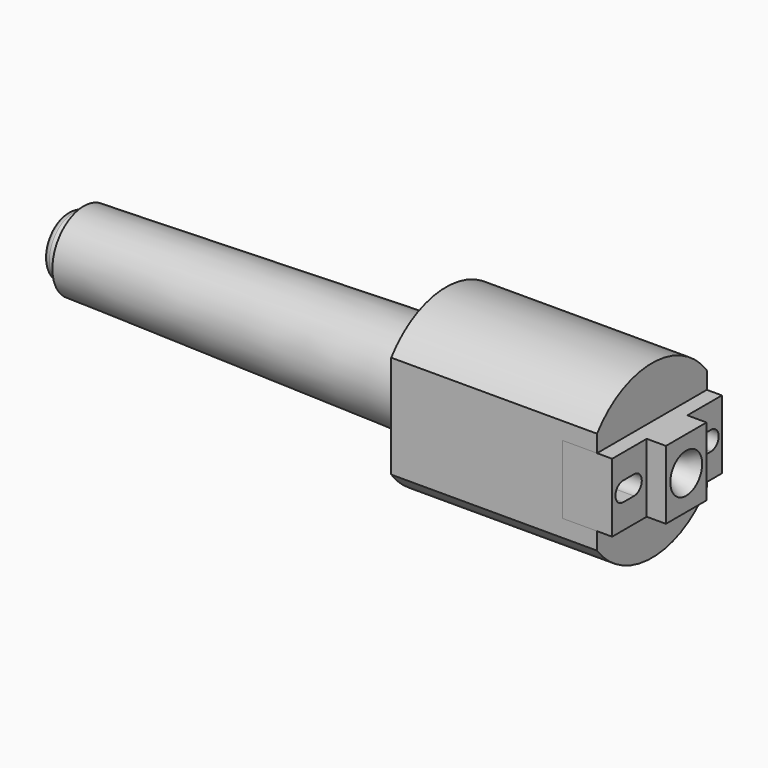
from build123d import *

# Parameters (mm, degrees)
F2_W      = 6.35
F2_H      = 12.7
F3_DEPTH  = 25.4
F6_DEPTH  = 38.1
F8_D      = 2.7051
F8_DEPTH  = 19.05
F8_TIP    = 0.8126940303
F9_DEPTH  = 12.7
F11_DEPTH = 25.4
F13_W     = 8.001
F13_H     = 12.7
F14_DEPTH = 3.556


# Not quite as in the source:
# - a feature names something its author has since deleted; it is built from what else it names


with BuildPart() as f1:
    # F0 (on Front) → F1 (revolve)
    with BuildSketch(Plane.XZ):
        Polygon((0, 5.588), (0, 0), (65.024, 0), (65.024, 8.89), (0, 7.2659854949), align=None)
        with BuildLine():
            Line((-3.175, 0), (0, 0))
            Line((0, 0), (0, 5.588))
            Line((0, 5.588), (-1.905, 5.588))
            ThreePointArc((-1.905, 5.588), (-2.8030256121, 5.2160256121), (-3.175, 4.318))
            Line((-3.175, 4.318), (-3.175, 0))
        make_face()
        with BuildLine():
            Line((65.024, 8.89), (65.024, 0))
            Line((65.024, 0), (67.056, 0))
            Line((67.056, 0), (67.056, 8.89))
            ThreePointArc((67.056, 8.89), (66.04, 8.5019225326), (65.024, 8.89))
        make_face()
        with BuildLine():
            Line((67.056, 8.89), (67.056, 0))
            Line((67.056, 0), (105.156, 0))
            Line((105.156, 0), (105.156, 15.875))
            Line((105.156, 15.875), (67.056, 15.875))
            Line((67.056, 15.875), (67.056, 11.1618450651))
            ThreePointArc((67.056, 11.1618450651), (67.4312152961, 10.6480929272), (67.564, 10.0259225326))
            ThreePointArc((67.564, 10.0259225326), (67.4312152961, 9.4037521379), (67.056, 8.89))
        make_face()
        with BuildLine():
            Line((67.056, 11.1618450651), (67.056, 8.89))
            ThreePointArc((67.056, 8.89), (67.4312152961, 9.4037521379), (67.564, 10.0259225326))
            ThreePointArc((67.564, 10.0259225326), (67.4312152961, 10.6480929272), (67.056, 11.1618450651))
        make_face()
    revolve(axis=Axis((32.512, 0, 0), (1, 0, 0)))

    # F2 (on Front) → F3 (cut, symmetric)
    with BuildSketch(Plane.XZ):
        with Locations((101.981, 0)):
            Rectangle(F2_W, F2_H)
    extrude(amount=F3_DEPTH, both=True, mode=Mode.SUBTRACT)

    # F4 (on face) → F6 (cut)
    with BuildSketch(Plane.YZ.offset(105.156)):
        with BuildLine():
            Line((-12.7, 6.35), (-14.5496778315, 6.35))
            ThreePointArc((-14.5496778315, 6.35), (-15.875, 0), (-14.5496778315, -6.35))
            ThreePointArc((-14.5496778315, -6.35), (-13.7170110348, -7.9911972363), (-12.7, -9.525))
            Line((-12.7, -9.525), (-12.7, 6.35))
        make_face()
        with BuildLine():
            ThreePointArc((-12.7, 9.525), (-13.7170110348, 7.9911972363), (-14.5496778315, 6.35))
            Line((-14.5496778315, 6.35), (-12.7, 6.35))
            Line((-12.7, 6.35), (-12.7, 9.525))
        make_face()
        with BuildLine():
            Line((14.5496778315, 6.35), (12.7, 6.35))
            Line((12.7, 6.35), (12.7, -9.525))
            ThreePointArc((12.7, -9.525), (13.7170110348, -7.9911972363), (14.5496778315, -6.35))
            ThreePointArc((14.5496778315, -6.35), (15.875, 0), (14.5496778315, 6.35))
        make_face()
        with BuildLine():
            Line((12.7, 9.525), (12.7, 6.35))
            Line((12.7, 6.35), (14.5496778315, 6.35))
            ThreePointArc((14.5496778315, 6.35), (13.7170110348, 7.9911972363), (12.7, 9.525))
        make_face()
    extrude(amount=-F6_DEPTH, mode=Mode.SUBTRACT)

    # F8
    with Locations(Plane.YZ.offset(98.806)):
        with Locations((-8.89, 0), (8.89, 0)):
            Hole(F8_D / 2, depth=F8_DEPTH)
            with Locations((0, 0, -(F8_DEPTH + F8_TIP / 2))):  # 118° drill point
                Cone(0, F8_D / 2, F8_TIP, mode=Mode.SUBTRACT)


with BuildPart() as f9:
    # F5 (on Front) → F9 (new body, symmetric)
    with BuildSketch(Plane.XZ):
        Polygon((98.806, 6.35), (98.806, -6.35), (111.506, -6.35), (111.506, -3.683), (111.506, 0), (103.9612241254, 0), (104.7014875327, 1.5875), (107.8764875327, 1.5875), (111.506, 3.683), (111.506, 6.35), align=None)
        Polygon((103.9612241254, 0), (111.506, 0), (111.506, 3.683), (107.8764875327, 1.5875), (104.7014875327, 1.5875), align=None)
    extrude(amount=F9_DEPTH, both=True)

    # F10 (on face) → F11 (cut)
    with BuildSketch(Plane.YZ.offset(111.506)):
        with BuildLine():
            ThreePointArc((7.62, 1.778), (5.842, 0), (7.62, -1.778))
            Line((7.62, -1.778), (10.16, -1.778))
            ThreePointArc((10.16, -1.778), (11.938, 0), (10.16, 1.778))
            Line((10.16, 1.778), (7.62, 1.778))
        make_face()
        with BuildLine():
            ThreePointArc((-10.16, 1.778), (-11.938, 0), (-10.16, -1.778))
            Line((-10.16, -1.778), (-7.62, -1.778))
            ThreePointArc((-7.62, -1.778), (-5.842, 0), (-7.62, 1.778))
            Line((-7.62, 1.778), (-10.16, 1.778))
        make_face()
    extrude(amount=-F11_DEPTH, mode=Mode.SUBTRACT)

    # F5 (on Front) → F12 (revolve, cut)
    with BuildSketch(Plane.XZ):
        Polygon((103.9612241254, 0), (111.506, 0), (111.506, 3.683), (107.8764875327, 1.5875), (104.7014875327, 1.5875), align=None)
    revolve(axis=Axis((107.7336120627, 0, 0), (1, 0, 0)), mode=Mode.SUBTRACT)

    # F13 (on face) → F14 (cut)
    with BuildSketch(Plane.YZ.offset(111.506)):
        with Locations((8.6995, 0)):
            Rectangle(F13_W, F13_H)
        with BuildLine():
            ThreePointArc((7.62, -1.778), (5.842, 0), (7.62, 1.778))
            Line((7.62, 1.778), (10.16, 1.778))
            ThreePointArc((10.16, 1.778), (11.938, 0), (10.16, -1.778))
            Line((10.16, -1.778), (7.62, -1.778))
        make_face(mode=Mode.SUBTRACT)
        with Locations((-8.6995, 0)):
            Rectangle(F13_W, F13_H)
        with BuildLine():
            Line((-7.62, -1.778), (-10.16, -1.778))
            ThreePointArc((-10.16, -1.778), (-11.938, 0), (-10.16, 1.778))
            Line((-10.16, 1.778), (-7.62, 1.778))
            ThreePointArc((-7.62, 1.778), (-5.842, 0), (-7.62, -1.778))
        make_face(mode=Mode.SUBTRACT)
    extrude(amount=-F14_DEPTH, mode=Mode.SUBTRACT)


with BuildPart() as f16:
    # F15 (on Front) → F16 (revolve)
    with BuildSketch(Plane.XZ):
        with BuildLine():
            Line((-3.175, 0), (3.175, 0))
            ThreePointArc((3.175, 0), (0, 3.175), (-3.175, 0))
        make_face()
    revolve(axis=Axis((0, 0, 0), (1, 0, 0)))


solid = Compound([f1.part, f9.part, f16.part])
